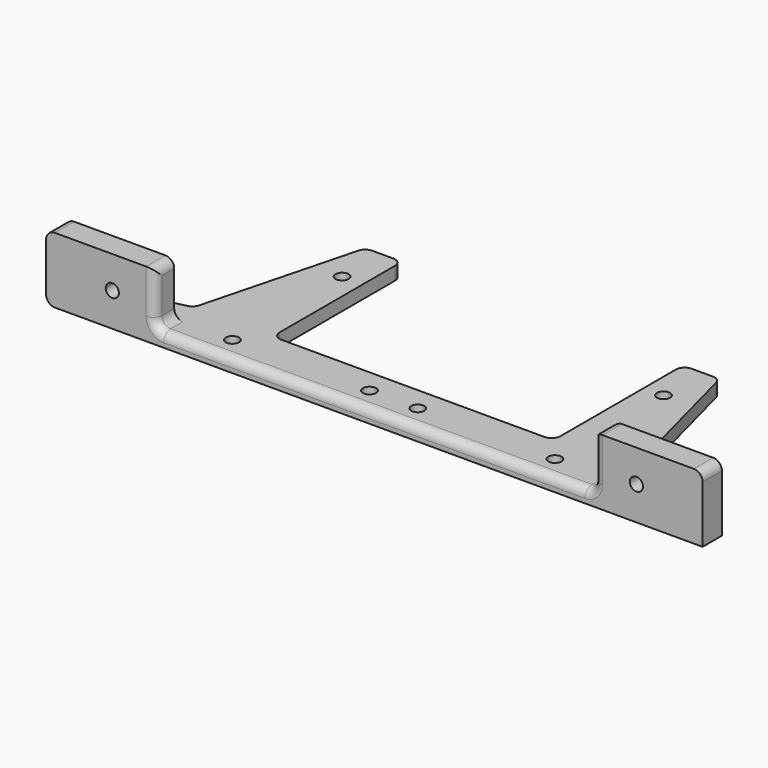
from build123d import *

# Parameters (mm, degrees)
F0_R     = 1.5
F1_DEPTH = 3
F0_W     = 24.7978687286
F0_H     = 5.5
F2_DEPTH = 15
F4_DEPTH = 25
F5_R     = 2


with BuildPart() as f1:
    # F0 (on Top) → F1 (new body)
    with BuildSketch(Plane.XY):
        Polygon((-40.3468825607, 42.3847011557), (-50, 5.5), (-31.9979505539, 5.5), (-31.9979505539, 42.3847011557), align=None)
        with Locations((-36.75, 31.25)):
            Circle(F0_R, mode=Mode.SUBTRACT)
        Polygon((-31.9979505539, 5.5), (-50, 5.5), (-50, 0), (-50, -5.5), (50, -5.5), (50, 0), (50, 5.5), (31.9979505539, 5.5), align=None)
        with Locations((-36.75, 0)):
            Circle(F0_R, mode=Mode.SUBTRACT)
        with Locations((-5.5, 0)):
            Circle(F0_R, mode=Mode.SUBTRACT)
        with Locations((5.5, 0)):
            Circle(F0_R, mode=Mode.SUBTRACT)
        with Locations((36.75, 0)):
            Circle(F0_R, mode=Mode.SUBTRACT)
        Polygon((31.9979505539, 42.3847011557), (31.9979505539, 5.5), (50, 5.5), (40.3468825607, 42.3847011557), align=None)
        with Locations((36.4979505539, 31.25)):
            Circle(F0_R, mode=Mode.SUBTRACT)
        Polygon((-50, 0), (-50, 5.5), (-74.7978687286, 0), align=None)
        Polygon((74.7978687286, 0), (50, 5.5), (50, 0), align=None)
    extrude(amount=F1_DEPTH)

    # F0 (on Top) → F2 (join)
    with BuildSketch(Plane.XY):
        with Locations((-62.3989343643, -2.75)):
            Rectangle(F0_W, F0_H)
        with Locations((62.3989343643, -2.75)):
            Rectangle(F0_W, F0_H)
    extrude(amount=F2_DEPTH)

    # F3 (on Front) → F4 (cut)
    with BuildSketch(Plane.XZ):
        with BuildLine():
            ThreePointArc((61.2087257832, 7.6567151021), (61.2088015755, 7.6654206983), (61.2088268399, 7.6741265878))
            ThreePointArc((61.2088268399, 7.6741265878), (58.2088521043, 7.6828324773), (61.2087257832, 7.6567151021))
        make_face()
        with BuildLine():
            ThreePointArc((-61.2087257832, 7.6567151021), (-59.7001209505, 6.1741518522), (-58.2088268399, 7.6741265878))
            ThreePointArc((-58.2088268399, 7.6741265878), (-59.7175327294, 9.1741013234), (-61.2087257832, 7.6567151021))
        make_face()
    extrude(amount=F4_DEPTH, mode=Mode.SUBTRACT)

    # F5
    f5_edges = [f1.edges().sort_by_distance(p)[0] for p in [
        (50, 5.5, 1.5),
        (40.346883, 42.384701, 1.5),
        (31.997951, 42.384701, 1.5),
        (31.997951, 5.5, 1.5),
        (-31.997951, 5.5, 1.5),
        (-31.997951, 42.384701, 1.5),
        (-40.346883, 42.384701, 1.5),
        (-50, 5.5, 1.5),
        (-74.797869, -2.75, 15),
        (-50, -2.75, 15),
        (-50, -2.75, 3),
        (-74.797869, -2.75, 0),
        (50, -2.75, 3),
        (50, -5.5, 9),
        (50, -2.75, 15),
        (50, 0, 9),
        (74.797869, -2.75, 15),
        (0, -5.5, 3),
        (62.398934, 0, 3),
        (-50, -5.5, 9),
    ]]
    fillet(f5_edges, radius=F5_R)


solid = f1.part
